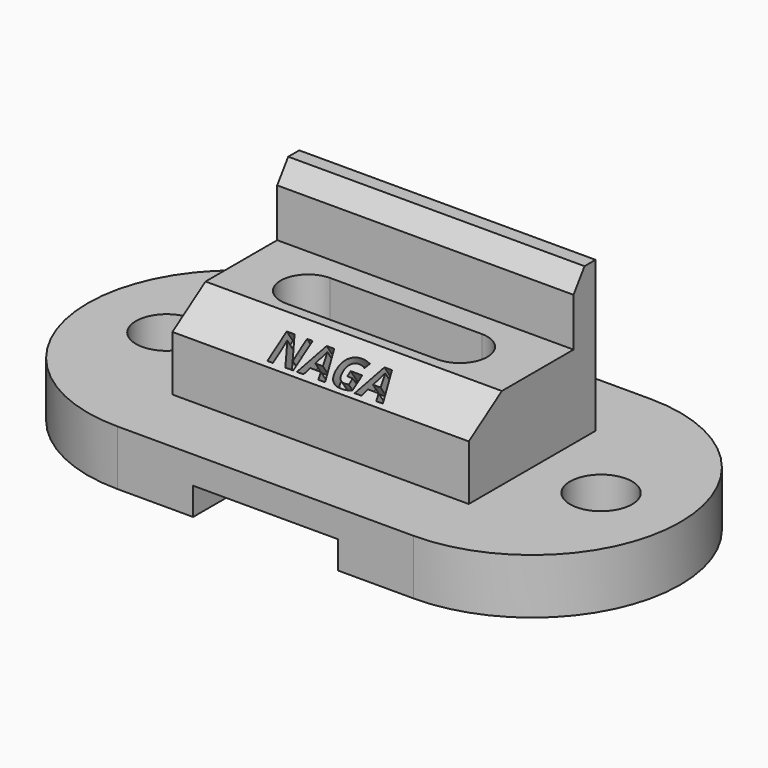
from build123d import *

# Parameters (mm, degrees)
F0_W         = 43
F0_H         = 43
F0_R         = 4.5
F1_DEPTH     = 8
F2_W         = 21
F2_H         = 4
F3_DEPTH     = 43
F6_DEPTH     = 21.5
F7_W         = 22
F7_H         = 8
F8_DEPTH     = 16
F9_TEXT_SIZE = 5.9279923638
F10_DEPTH    = 2


# Not quite as in the source:
# - Text() gives the source's letters only with a copy of the font that has no kerning and outlines rounded to 1/6400 em; it was checked with that copy


with BuildPart() as f1:
    # F0 (on Top) → F1 (new body)
    with BuildSketch(Plane.XY):
        Rectangle(F0_W, F0_H)
        with BuildLine():
            Line((21.5, 21.5), (21.5, -21.5))
            ThreePointArc((21.5, -21.5), (43, 0), (21.5, 21.5))
        make_face()
        with Locations((31.5, 0)):
            Circle(F0_R, mode=Mode.SUBTRACT)
        with BuildLine():
            ThreePointArc((-21.5, 21.5), (-43, 0), (-21.5, -21.5))
            Line((-21.5, -21.5), (-21.5, 21.5))
        make_face()
        with Locations((-31.5, 0)):
            Circle(F0_R, mode=Mode.SUBTRACT)
    extrude(amount=F1_DEPTH)

    # F2 (on face) → F3 (cut)
    with BuildSketch(Plane.XZ.offset(21.5)):
        with Locations((0, 2)):
            Rectangle(F2_W, F2_H)
    extrude(amount=-F3_DEPTH, mode=Mode.SUBTRACT)

    # F5 (on Right) → F6 (join, symmetric)
    with BuildSketch(Plane.YZ):
        Polygon((-11.5, 16), (-11.5, 8), (11.5, 8), (11.5, 29.8476405442), (9.5, 29.8476405442), (7.5, 27), (7.5, 20), (-5.5, 20), align=None)
    extrude(amount=F6_DEPTH, both=True)

    # F7 (on face) → F8 (cut)
    with BuildSketch(Plane.XY.offset(20)):
        Rectangle(F7_W, F7_H)
        with BuildLine():
            Line((11, 4), (11, -4))
            ThreePointArc((11, -4), (15, 0), (11, 4))
        make_face()
        with BuildLine():
            ThreePointArc((-11, 4), (-15, 0), (-11, -4))
            Line((-11, -4), (-11, 4))
        make_face()
    extrude(amount=-F8_DEPTH, mode=Mode.SUBTRACT)

    # F9 (on face) → F10 (cut)
    with BuildSketch(Plane(origin=(0, -10.9230769231, 16.3846153846), x_dir=(1, 0, 0), z_dir=(0, -0.5547001962, 0.8320502943))):
        with Locations((-8.7224766612, 0)):
            Text('NAGA', F9_TEXT_SIZE, font='Open Sans', font_style=FontStyle.BOLD, text_align=(TextAlign.LEFT, TextAlign.BOTTOM))
    extrude(amount=-F10_DEPTH, mode=Mode.SUBTRACT)


solid = f1.part
